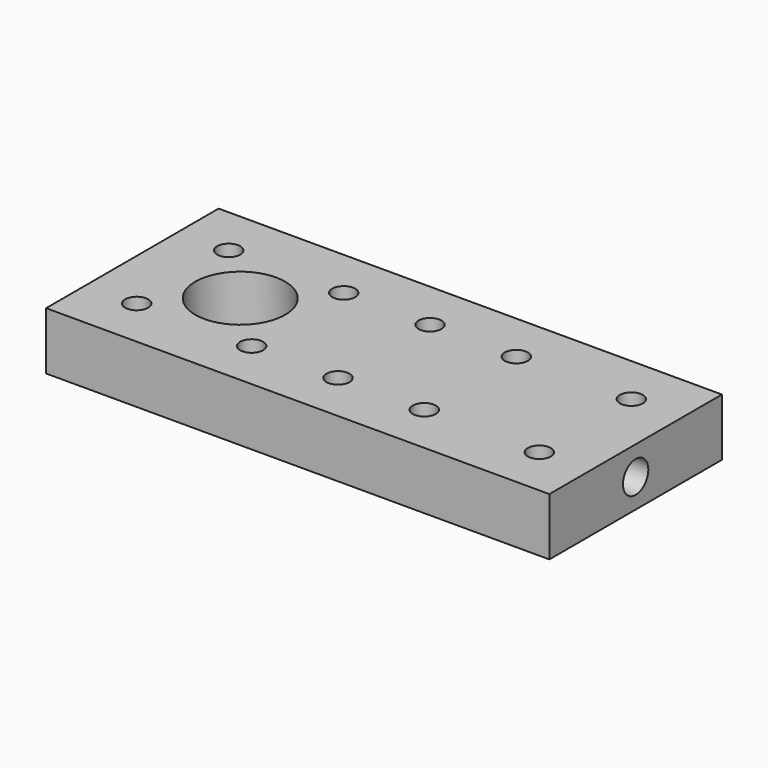
from build123d import *

# Parameters (mm, degrees)
F0_W     = 70
F0_H     = 30
F1_DEPTH = 8
F2_D     = 3.2
F3_D     = 12.5
F5_D     = 3.5
F5_DEPTH = 50
F5_TIP   = 1.0515060833
F6_D     = 4.4
F6_DEPTH = 15
F6_TIP   = 1.3218933619
F7_R     = 1.7108756352
F8_DEPTH = 3.456151576


with BuildPart() as f1:
    # F0 (on Top) → F1 (new body)
    with BuildSketch(Plane.XY):
        Rectangle(F0_W, F0_H)
    extrude(amount=-F1_DEPTH)

    # F2 (through all)
    with Locations(Plane.XY):
        with Locations((-28, 8), (-12, 8), (-28, -8), (-12, -8), (0, 8), (0, -8), (12, 8), (12, -8), (28, 8), (28, -8)):
            Hole(F2_D / 2)

    # F3 (through all)
    with Locations(Plane.XY):
        with Locations((-20, 0)):
            Hole(F3_D / 2)

    # F5
    with Locations(Plane.YZ.offset(35)):
        with Locations((0, -4)):
            Hole(F5_D / 2, depth=F5_DEPTH)
            with Locations((0, 0, -(F5_DEPTH + F5_TIP / 2))):  # 118° drill point
                Cone(0, F5_D / 2, F5_TIP, mode=Mode.SUBTRACT)

    # F6
    with Locations(Plane.YZ.offset(35)):
        with Locations((0, -4)):
            Hole(F6_D / 2, depth=F6_DEPTH)
            with Locations((0, 0, -(F6_DEPTH + F6_TIP / 2))):  # 118° drill point
                Cone(0, F6_D / 2, F6_TIP, mode=Mode.SUBTRACT)

    # F7 (on face) → F8 (cut, through all)
    with BuildSketch(Plane(origin=(0, 0, -8), x_dir=(1, 0, 0), z_dir=(0, 0, -1))):
        with Locations((20.1314277947, 0)):
            Circle(F7_R)
    extrude(amount=-F8_DEPTH, mode=Mode.SUBTRACT)


solid = f1.part
